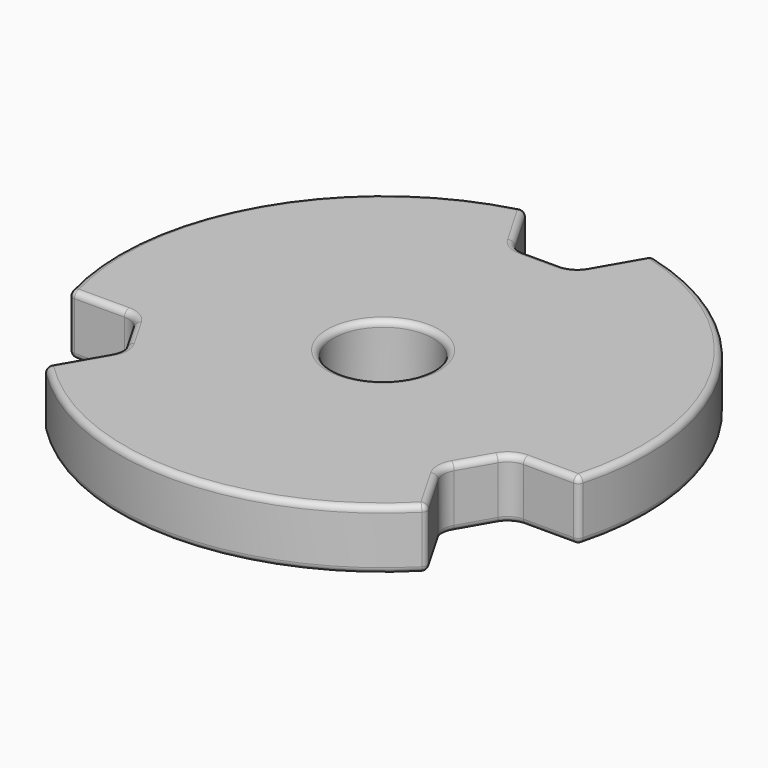
from build123d import *

# Parameters (mm, degrees)
F0_W     = 10.75
F0_H     = 3
F3_DEPTH = 25
F4_R     = 1
F5_R     = 0.3


# Not quite as in the source:
# - a feature names something its author has since deleted; it is built from what else it names


with BuildPart() as f1:
    # F0 (on Front) → F1 (revolve)
    with BuildSketch(Plane.XZ):
        with Locations((7.875, -1.5)):
            Rectangle(F0_W, F0_H)
    revolve(axis=Axis((0, 0, -1.5), (0, 0, -1)))

    # F2 (on face) → F3 (cut)
    with BuildSketch(Plane.XY):
        with BuildLine():
            Line((1.5, 10), (3.1561892964, 12.8686040084))
            ThreePointArc((3.1561892964, 12.8686040084), (0, 13.25), (-3.1561892964, 12.8686040084))
            Line((-3.1561892964, 12.8686040084), (-1.5, 10))
            Line((-1.5, 10), (1.5, 10))
        make_face()
        with BuildLine():
            ThreePointArc((-12.7226326307, -3.7009618943), (-11.4748366001, -6.625), (-9.5664433343, -9.1676421141))
            Line((-9.5664433343, -9.1676421141), (-7.9102540378, -6.2990381057))
            Line((-7.9102540378, -6.2990381057), (-9.4102540378, -3.7009618943))
            Line((-9.4102540378, -3.7009618943), (-12.7226326307, -3.7009618943))
        make_face()
        with BuildLine():
            ThreePointArc((9.5664433343, -9.1676421141), (11.4748366001, -6.625), (12.7226326307, -3.7009618943))
            Line((12.7226326307, -3.7009618943), (9.4102540378, -3.7009618943))
            Line((9.4102540378, -3.7009618943), (7.9102540378, -6.2990381057))
            Line((7.9102540378, -6.2990381057), (9.5664433343, -9.1676421141))
        make_face()
    extrude(amount=-F3_DEPTH, mode=Mode.SUBTRACT)

    # F4
    f4_edges = [f1.edges().sort_by_distance(p)[0] for p in [
        (-9.410254, -3.700962, -1.5),
        (-7.910254, -6.299038, -1.5),
        (7.910254, -6.299038, -1.5),
        (9.410254, -3.700962, -1.5),
        (1.5, 10, -1.5),
        (-1.5, 10, -1.5),
    ]]
    fillet(f4_edges, radius=F4_R)

    # F5
    f5_edges = [f1.edges().sort_by_distance(p)[0] for p in [
        (2.472432, 11.684302, 0),
        (1.42265, 10.133975, 0),
        (11.474837, 6.625, 0),
        (0, 10, 0),
        (11.355118, -3.700962, 0),
        (-1.42265, 10.133975, 0),
        (9.487604, -3.834936, 0),
        (-2.472432, 11.684302, 0),
        (8.660254, -5, 0),
        (-11.474837, 6.625, 0),
        (8.064955, -6.299038, 0),
        (-11.355118, -3.700962, 0),
        (8.882686, -7.98334, 0),
        (-9.487604, -3.834936, 0),
        (0, -13.25, 0),
        (-8.660254, -5, 0),
        (-8.882686, -7.98334, 0),
        (-8.064955, -6.299038, 0),
        (-2.5, 0, 0),
        (12.722633, -3.700962, -1.5),
        (9.566443, -9.167642, -1.5),
        (-9.566443, -9.167642, -1.5),
        (-12.722633, -3.700962, -1.5),
        (2.472432, 11.684302, -3),
        (1.42265, 10.133975, -3),
        (11.474837, 6.625, -3),
        (0, 10, -3),
        (11.355118, -3.700962, -3),
        (-1.42265, 10.133975, -3),
        (9.487604, -3.834936, -3),
        (-2.472432, 11.684302, -3),
        (8.660254, -5, -3),
        (-11.474837, 6.625, -3),
        (8.064955, -6.299038, -3),
        (-11.355118, -3.700962, -3),
        (8.882686, -7.98334, -3),
        (-9.487604, -3.834936, -3),
        (0, -13.25, -3),
        (-8.660254, -5, -3),
        (-8.882686, -7.98334, -3),
        (-8.064955, -6.299038, -3),
        (-2.5, 0, -3),
        (-3.156189, 12.868604, -1.5),
        (3.156189, 12.868604, -1.5),
    ]]
    fillet(f5_edges, radius=F5_R)


solid = f1.part
